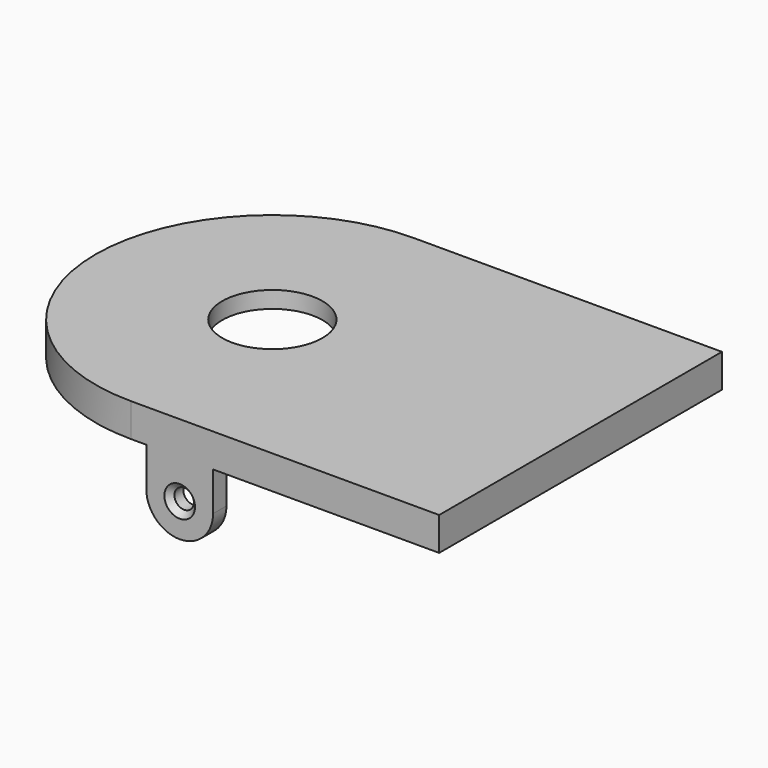
from build123d import *

# Parameters (mm, degrees)
F0_R     = 9
F1_DEPTH = 3
F3_DEPTH = 3
F4_R     = 1.75
F5_DEPTH = 3
F7_SIZE  = 1


# Not quite as in the source:
# - a feature names something its author has since deleted; it is built from what else it names


with BuildPart() as f1:
    # F0 (on Top) → F1 (new body)
    with BuildSketch(Plane.XY):
        with BuildLine():
            Line((55.375, -31.75), (55.375, 31.75))
            Line((55.375, 31.75), (0, 31.75))
            ThreePointArc((0, 31.75), (-31.75, 0), (0, -31.75))
            Line((0, -31.75), (55.375, -31.75))
        make_face()
        Circle(F0_R, mode=Mode.SUBTRACT)
    extrude(amount=F1_DEPTH)

    # F2 (on face) → F3 (join)
    with BuildSketch(Plane(origin=(0, 0, 0), x_dir=(1, 0, 0), z_dir=(0, 0, -1))):
        with BuildLine():
            ThreePointArc((0, 31.75), (-31.75, 0), (0, -31.75))
            Line((0, -31.75), (55.375, -31.75))
            Line((55.375, -31.75), (55.375, 31.75))
            Line((55.375, 31.75), (0, 31.75))
        make_face()
        with BuildLine():
            Line((52.375, -28.75), (0, -28.75))
            ThreePointArc((0, -28.75), (-28.75, 0), (0, 28.75))
            Line((0, 28.75), (52.375, 28.75))
            Line((52.375, 28.75), (52.375, -28.75))
        make_face(mode=Mode.SUBTRACT)
    extrude(amount=F3_DEPTH)

    # F4 (on face) → F5 (join)
    with BuildSketch(Plane.XZ.offset(31.75)):
        with BuildLine():
            Line((14.75, -3), (2.75, -3))
            Line((2.75, -3), (2.75, -10))
            ThreePointArc((2.75, -10), (8.75, -16), (14.75, -10))
            Line((14.75, -10), (14.75, -3))
        make_face()
        with Locations((8.75, -10)):
            Circle(F4_R, mode=Mode.SUBTRACT)
    extrude(amount=-F5_DEPTH)

    # F6: F1 across plane


with BuildPart() as f1_1:
    add(f1.part)
    add(f1.part.mirror(Plane.XZ))

    # F7
    f7_edges = [f1_1.edges().sort_by_distance(p)[0] for p in [
        (7, -31.75, -10),
        (7, 31.75, -10),
    ]]
    chamfer(f7_edges, length=F7_SIZE)


solid = f1_1.part
